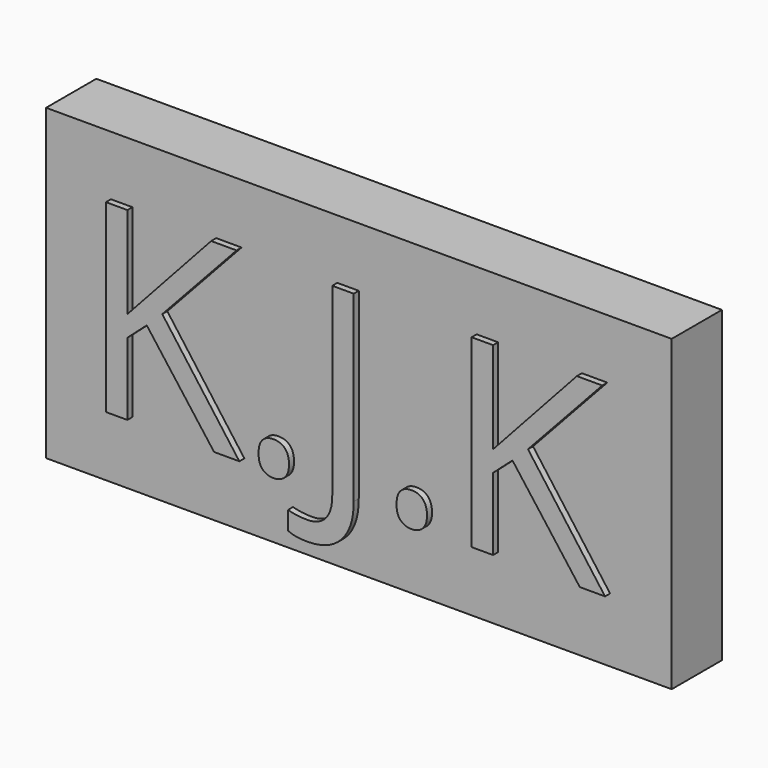
from build123d import *

# Parameters (mm, degrees)
F0_W         = 99.6437892318
F0_H         = 49.1305626929
F1_DEPTH     = 10
F2_TEXT_SIZE = 41.223790807
F3_DEPTH     = 1


# Not quite as in the source:
# - Text() gives the source's letters only with a copy of the font that has no kerning and outlines rounded to 1/6400 em; it was checked with that copy


with BuildPart() as f1:
    # F0 (on Front) → F1 (new body)
    with BuildSketch(Plane.XZ):
        with Locations((49.8218946159, 24.5652813464)):
            Rectangle(F0_W, F0_H)
    extrude(amount=F1_DEPTH)

    # F2 (on face) → F3 (join)
    with BuildSketch(Plane.XZ.offset(10)):
        with Locations((6.283425726, 10.2316942066)):
            Text('K.J.K', F2_TEXT_SIZE, font='Open Sans', text_align=(TextAlign.LEFT, TextAlign.BOTTOM))
    extrude(amount=F3_DEPTH)


solid = f1.part
